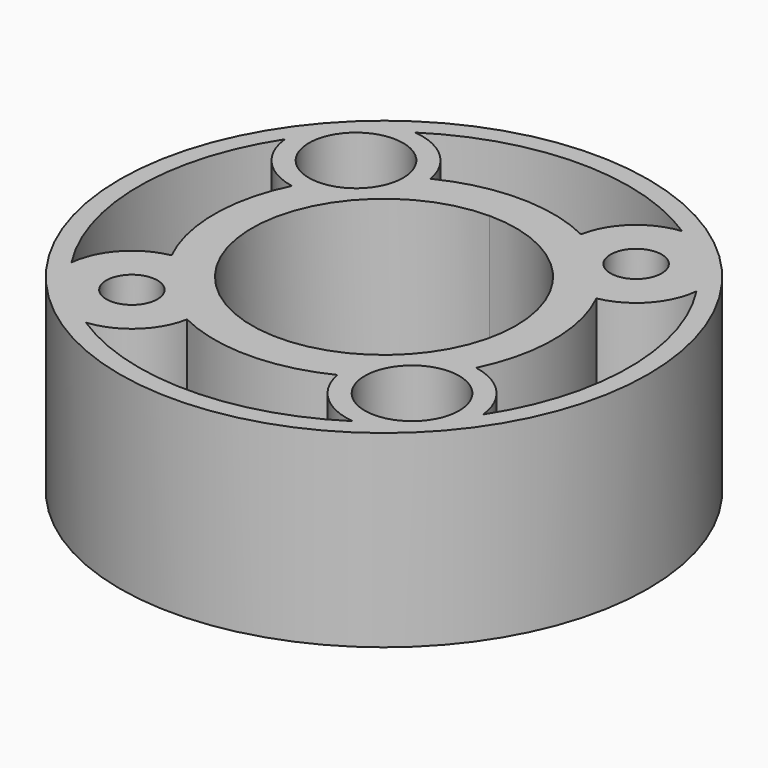
from build123d import *

# Parameters (mm, degrees)
F0_R            = 22.225
F0_R_2          = 2.15265
F1_DEPTH        = 15.875
F4_R            = 3.96875
F5_DEPTH        = 12.7
F6_R            = 3.96875
F7_DEPTH        = 12.7
F9_DEPTH        = 15.875
F9_COPIES_COUNT = 4


# Not quite as in the source:
# - a pattern or mirror of a feature is missing from the dataset's text; its kind, count and spacing are read off the source's solid


with BuildPart() as f1:
    # F0 (on Top) → F1 (new body)
    with BuildSketch(Plane.XY):
        Circle(F0_R)
        with Locations((-11.7865861589, -11.7865861589)):
            Circle(F0_R_2, mode=Mode.SUBTRACT)
        with Locations((11.7865861589, -11.7865861589)):
            Circle(F0_R_2, mode=Mode.SUBTRACT)
        with Locations((-11.7865861589, 11.7865861589)):
            Circle(F0_R_2, mode=Mode.SUBTRACT)
        with BuildLine():
            ThreePointArc((0, 11.1125), (7.8577241059, 7.8577241059), (11.1125, 0))
            ThreePointArc((11.1125, 0), (-7.8577241059, -7.8577241059), (0, 11.1125))
        make_face(mode=Mode.SUBTRACT)
        with Locations((11.7865861589, 11.7865861589)):
            Circle(F0_R_2, mode=Mode.SUBTRACT)
    extrude(amount=F1_DEPTH)

    # F4 (on face) → F5 (cut, through all)
    with BuildSketch(Plane(origin=(0, 0, 0), x_dir=(1, 0, 0), z_dir=(0, 0, -1))):
        with Locations((11.7865861589, -11.7865861589)):
            Circle(F4_R)
        with Locations((-11.7865861589, 11.7865861589)):
            Circle(F4_R)
    extrude(amount=-F5_DEPTH, mode=Mode.SUBTRACT)

    # F6 (on face) → F7 (cut, through all)
    with BuildSketch(Plane.XY.offset(15.875)):
        with Locations((-11.7865861589, 11.7865861589)):
            Circle(F6_R)
        with Locations((11.7865861589, -11.7865861589)):
            Circle(F6_R)
    extrude(amount=-F7_DEPTH, mode=Mode.SUBTRACT)

    # F8 (on face) → F9 (cut, through all)
    with BuildSketch(Plane(origin=(0, 0, 0), x_dir=(1, 0, 0), z_dir=(0, 0, -1))):
        with BuildLine():
            ThreePointArc((-11.229543123, 17.3148424047), (-8.0281867, 15.8788163052), (-6.3255746232, 12.8109235396))
            ThreePointArc((-6.3255746232, 12.8109235396), (0, 14.2875), (6.3255746232, 12.8109235396))
            ThreePointArc((6.3255746232, 12.8109235396), (8.0281867, 15.8788163052), (11.229543123, 17.3148424047))
            ThreePointArc((11.229543123, 17.3148424047), (0, 20.6375), (-11.229543123, 17.3148424047))
        make_face()
    f9 = extrude(amount=-F9_DEPTH, mode=Mode.SUBTRACT)

    # F9_copies: F9 ×4 about axis
    f9_copies_axis = Axis((0, 0, 0), (0, 0, 1))
    for i in range(1, F9_COPIES_COUNT):
        add(f9.rotate(f9_copies_axis, i * 360 / F9_COPIES_COUNT), mode=Mode.SUBTRACT)


solid = f1.part
